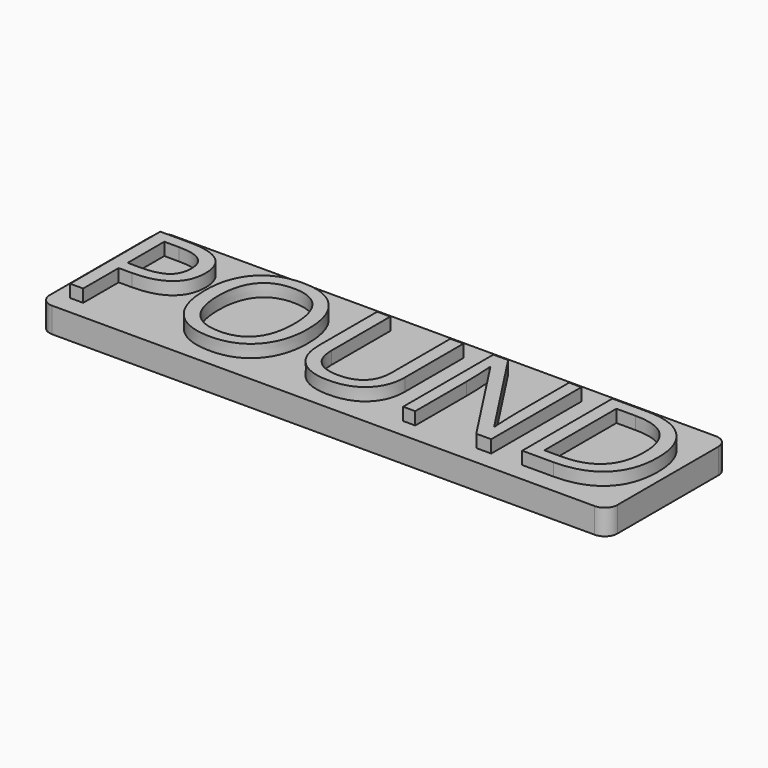
from build123d import *

# Parameters (mm, degrees)
F0_W         = 90
F0_H         = 24
F1_DEPTH     = 4
F2_R         = 2
F3_TEXT_SIZE = 25.0315066707
F4_DEPTH     = 2
F5_TEXT_SIZE = 17.3611111111
F6_DEPTH     = 1.5


# Not quite as in the source:
# - a feature names something its author has since deleted; it is built from what else it names
# - Text() gives the source's letters only with a copy of the font that has no kerning and outlines rounded to 1/6400 em; it was checked with that copy


with BuildPart() as f1:
    # F0 (on Top) → F1 (new body)
    with BuildSketch(Plane.XY):
        Rectangle(F0_W, F0_H)
    extrude(amount=F1_DEPTH)

    # F2
    f2_edges = [f1.edges().sort_by_distance(p)[0] for p in [
        (-45, -12, 2),
        (45, 12, 2),
        (-45, 12, 2),
        (45, -12, 2),
    ]]
    fillet(f2_edges, radius=F2_R)

    # F3 (on face) → F4 (join)
    with BuildSketch(Plane.XY.offset(4)):
        with Locations((-45, -9.0113424015)):
            Text('POUND', F3_TEXT_SIZE, font='Open Sans', text_align=(TextAlign.LEFT, TextAlign.BOTTOM))
    extrude(amount=F4_DEPTH)

    # F5 (on face) → F6 (cut)
    with BuildSketch(Plane(origin=(0, 0, 0), x_dir=(1, 0, 0), z_dir=(0, 0, -1))):
        with Locations((-41.3886176215, -6.25)):
            Text('16 ounces', F5_TEXT_SIZE, font='Open Sans', text_align=(TextAlign.LEFT, TextAlign.BOTTOM))
    extrude(amount=-F6_DEPTH, mode=Mode.SUBTRACT)


solid = f1.part
